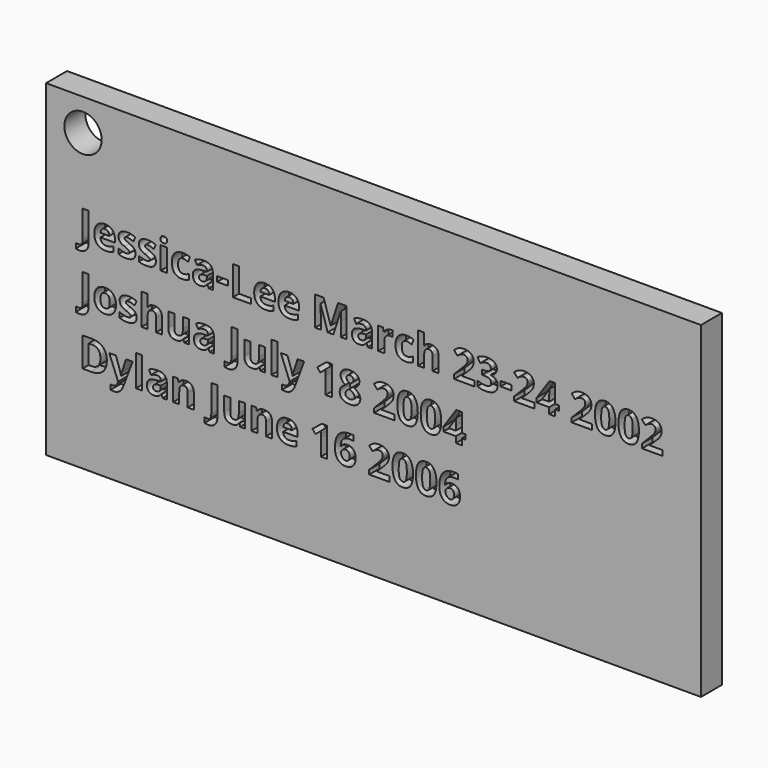
from build123d import *

# Parameters (mm, degrees)
F0_W         = 100
F0_H         = 50
F0_R         = 2.8498202562
F1_DEPTH     = 4
F2_TEXT_SIZE = 6.2696607199
F3_DEPTH     = 2


# Not quite as in the source:
# - Text() gives the source's letters only with a copy of the font that has no kerning and outlines rounded to 1/6400 em; it was checked with that copy


with BuildPart() as f1:
    # F0 (on Front) → F1 (new body)
    with BuildSketch(Plane.XZ):
        Rectangle(F0_W, F0_H)
        with Locations((-44.3621836603, 20.1387219131)):
            Circle(F0_R, mode=Mode.SUBTRACT)
    extrude(amount=F1_DEPTH)

    # F2 (on face) → F3 (cut)
    with BuildSketch(Plane.XZ.offset(4)):
        with Locations((-45, 5.4858442817)):
            Text('Jessica-Lee March 23-24 2002', F2_TEXT_SIZE, font='Open Sans', font_style=FontStyle.BOLD, text_align=(TextAlign.LEFT, TextAlign.BOTTOM))
        with Locations((-45, -3.0408942974)):
            Text('Joshua July 18 2004', F2_TEXT_SIZE, font='Open Sans', font_style=FontStyle.BOLD, text_align=(TextAlign.LEFT, TextAlign.BOTTOM))
        with Locations((-45, -11.5676328765)):
            Text('Dylan June 16 2006', F2_TEXT_SIZE, font='Open Sans', font_style=FontStyle.BOLD, text_align=(TextAlign.LEFT, TextAlign.BOTTOM))
    extrude(amount=-F3_DEPTH, mode=Mode.SUBTRACT)


solid = f1.part
